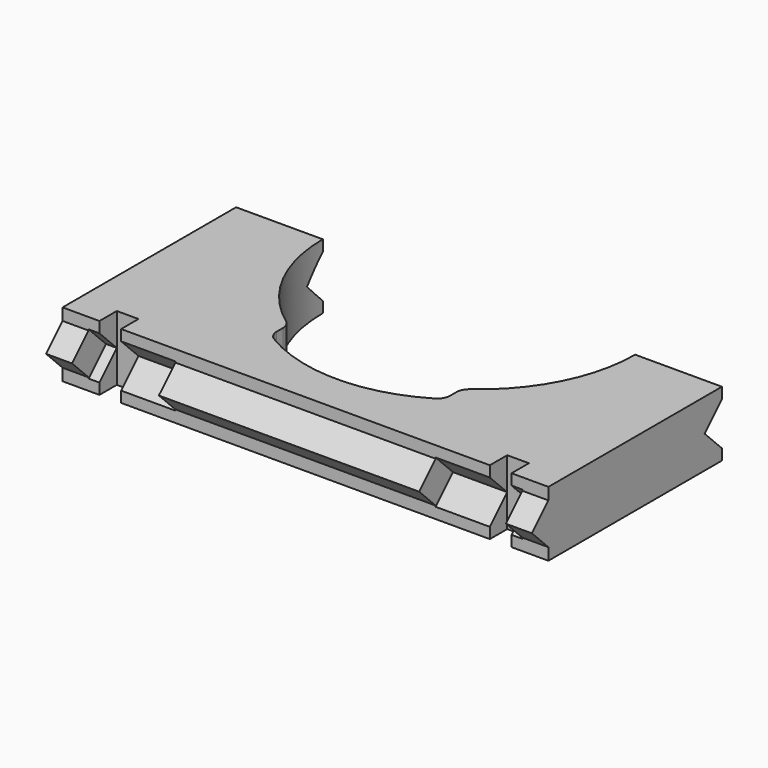
from build123d import *

# Parameters (mm, degrees)
F1_DEPTH       = 15
F3_DEPTH       = 112.001
F5_DEPTH       = 5
F7_DEPTH       = 112
F9_DEPTH       = 25
F12_DEPTH      = 15
F12_DEPTH_BACK = 5
F14_DEPTH      = 25
F15_R          = 3


# Not quite as in the source:
# - a pattern or mirror of a feature is missing from the dataset's text; its kind, count and spacing are read off the source's solid


with BuildPart() as f1:
    # F0 (on Top) → F1 (new body)
    with BuildSketch(Plane.XY):
        with BuildLine():
            Line((-56, 50), (-56, 0))
            Line((-56, 0), (56, 0))
            Line((56, 0), (56, 50))
            Line((56, 50), (36, 50))
            ThreePointArc((36, 50), (0, 14), (-36, 50))
            Line((-36, 50), (-56, 50))
        make_face()
    extrude(amount=F1_DEPTH)

    # F2 (on face) → F3 (cut, through all)
    with BuildSketch(Plane(origin=(-56, 0, 0), x_dir=(0, -1, 0), z_dir=(-1, 0, 0))):
        Polygon((-50, 12.5), (-50, 2.5), (-45, 7.5), align=None)
    extrude(amount=-F3_DEPTH, mode=Mode.SUBTRACT)

    # F4 (on face) → F5 (cut)
    with BuildSketch(Plane(origin=(0, 0, 0), x_dir=(1, 0, 0), z_dir=(0, 0, -1))):
        Polygon((-48.5, -45), (-48.5, -50), (-43.5, -50), (-43.5, -45), (-39.5, -41), (-52.5, -41), align=None)
        Polygon((43.5, -45), (43.5, -50), (48.5, -50), (48.5, -45), (52.5, -41), (39.5, -41), align=None)
    extrude(amount=-F5_DEPTH, mode=Mode.SUBTRACT)

    # F6 (on face) → F7 (join, through all)
    with BuildSketch(Plane(origin=(-56, 0, 0), x_dir=(0, -1, 0), z_dir=(-1, 0, 0))):
        Polygon((4.75, 7.5), (0, 12.25), (0, 2.75), align=None)
    extrude(amount=-F7_DEPTH)

    # F8 (on face) → F9 (cut)
    with BuildSketch(Plane(origin=(0, 0, 0), x_dir=(1, 0, 0), z_dir=(0, 0, -1))):
        Polygon((-47.5, 11.2829459831), (-47.5, 0), (-47.5, -5), (-42.5, -5), (-42.5, 0), (-42.5, 11.2829459831), align=None)
        Polygon((47.5, 11.2829459831), (42.5, 11.2829459831), (42.5, 0), (42.5, -5), (47.5, -5), (47.5, 0), align=None)
    extrude(amount=-F9_DEPTH, mode=Mode.SUBTRACT)

    # F11 (on mid) → F12 (cut, two sides)
    with BuildSketch(Plane(origin=(-45, 0, 0), x_dir=(0, -1, 0), z_dir=(-1, 0, 0))) as f12_sk:
        Polygon((0, 12.5), (-5, 7.5), (0, 2.5), (5, 7.5), align=None)
    f12 = extrude(amount=-F12_DEPTH, mode=Mode.SUBTRACT) + extrude(f12_sk.sketch, amount=F12_DEPTH_BACK, mode=Mode.SUBTRACT)

    # F12_copies: F12 across plane
    add(f12.mirror(Plane(origin=(0, 0, 0), x_dir=(0, 0, 1), z_dir=(1, 0, 0))), mode=Mode.SUBTRACT)

    # F13 (on face) → F14 (cut)
    with BuildSketch(Plane.XY.offset(15)):
        with BuildLine():
            Line((20, 15.0667409058), (20, 20.0667409058))
            ThreePointArc((20, 20.0667409058), (0, 14), (-20, 20.0667409058))
            Line((-20, 20.0667409058), (-20, 15.0667409058))
            ThreePointArc((-20, 15.0667409058), (0, 9), (20, 15.0667409058))
        make_face()
    extrude(amount=-F14_DEPTH, mode=Mode.SUBTRACT)

    # F15
    f15_edges = [f1.edges().sort_by_distance(p)[0] for p in [
        (-20, 20.066741, 7.5),
        (20, 20.066741, 7.5),
        (-20, 15.066741, 7.5),
        (20, 15.066741, 7.5),
    ]]
    fillet(f15_edges, radius=F15_R)


solid = f1.part
